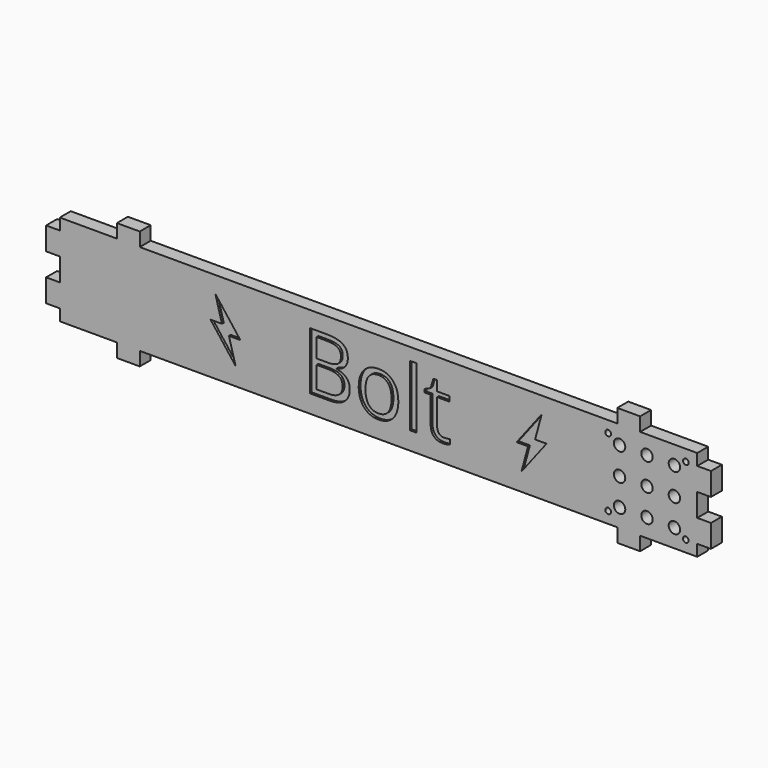
from build123d import *

# Parameters (mm, degrees)
F0_R         = 1.25
F0_R_2       = 2.5
F1_DEPTH     = 6
F3_TEXT_SIZE = 35.2573791761
F4_DEPTH     = 1


# Not quite as in the source:
# - a feature names something its author has since deleted; it is built from what else it names
# - Text() gives the source's letters only with a copy of the font that has no kerning and outlines rounded to 1/6400 em; it was checked with that copy


with BuildPart() as f1:
    # F0 (on Front) → F1 (new body)
    with BuildSketch(Plane.XZ):
        Polygon((-139.5, -63.528323397), (-139.5, -68.528323397), (-114.5, -68.528323397), (-114.5, -74.528323397), (-104.5, -74.528323397), (-104.5, -68.528323397), (0, -68.528323397), (104.5, -68.528323397), (104.5, -74.528323397), (114.5, -74.528323397), (114.5, -68.528323397), (139.5, -68.528323397), (139.5, -63.528323397), (145.5, -63.528323397), (145.5, -53.528323397), (139.5, -53.528323397), (139.5, -43.528323397), (145.5, -43.528323397), (145.5, -33.5283233315), (139.5, -33.5283233315), (139.4991906481, -28.528323397), (114.4991906481, -28.528323397), (114.4991906481, -22.528323397), (104.4991906481, -22.528323397), (104.4991906481, -28.528323397), (0, -28.528323397), (-104.4991906481, -28.528323397), (-104.4991906481, -22.528323397), (-114.4991906481, -22.528323397), (-114.4991906481, -28.528323397), (-139.4991906481, -28.528323397), (-139.5, -33.5283233315), (-145.5, -33.5283233315), (-145.5, -43.528323397), (-139.5, -43.528323397), (-139.5, -53.528323397), (-145.5, -53.528323397), (-145.5, -63.528323397), align=None)
        with Locations((100.5, -63.528323397)):
            Circle(F0_R, mode=Mode.SUBTRACT)
        with Locations((134.5, -63.528323397)):
            Circle(F0_R, mode=Mode.SUBTRACT)
        with Locations((105.5, -60.528323397)):
            Circle(F0_R_2, mode=Mode.SUBTRACT)
        with Locations((117.5, -60.528323397)):
            Circle(F0_R_2, mode=Mode.SUBTRACT)
        with Locations((129.5, -60.528323397)):
            Circle(F0_R_2, mode=Mode.SUBTRACT)
        with Locations((105.5, -48.528323397)):
            Circle(F0_R_2, mode=Mode.SUBTRACT)
        with Locations((117.5, -48.528323397)):
            Circle(F0_R_2, mode=Mode.SUBTRACT)
        with Locations((129.5, -48.528323397)):
            Circle(F0_R_2, mode=Mode.SUBTRACT)
        with Locations((105.5, -36.528323397)):
            Circle(F0_R_2, mode=Mode.SUBTRACT)
        with Locations((117.5, -36.528323397)):
            Circle(F0_R_2, mode=Mode.SUBTRACT)
        with Locations((129.5, -36.528323397)):
            Circle(F0_R_2, mode=Mode.SUBTRACT)
        with Locations((100.5, -33.528323397)):
            Circle(F0_R, mode=Mode.SUBTRACT)
        with Locations((134.5, -33.528323397)):
            Circle(F0_R, mode=Mode.SUBTRACT)
    extrude(amount=F1_DEPTH)

    # F3 (on offset) → F4 (cut)
    with BuildSketch(Plane.XZ.offset(6)):
        Polygon((65.4577315602, -50.0641831515), (62.5708529191, -60.6786040831), (73.5300201305, -46.3993655168), (68.5300201305, -46.3993655168), (71.4168987715, -35.7849445852), (60.4577315602, -50.0641831515), align=None)
        Polygon((-60.4577315602, -50.0641831515), (-71.4168987715, -35.7849445852), (-68.5300201305, -46.3993655168), (-73.5300201305, -46.3993655168), (-62.5708529191, -60.6786040831), (-65.4577315602, -50.0641831515), align=None)
        with Locations((-33.4915327727, -60.6786040831)):
            Text('Bolt', F3_TEXT_SIZE, font='Open Sans', text_align=(TextAlign.LEFT, TextAlign.BOTTOM))
    extrude(amount=-F4_DEPTH, mode=Mode.SUBTRACT)


solid = f1.part
